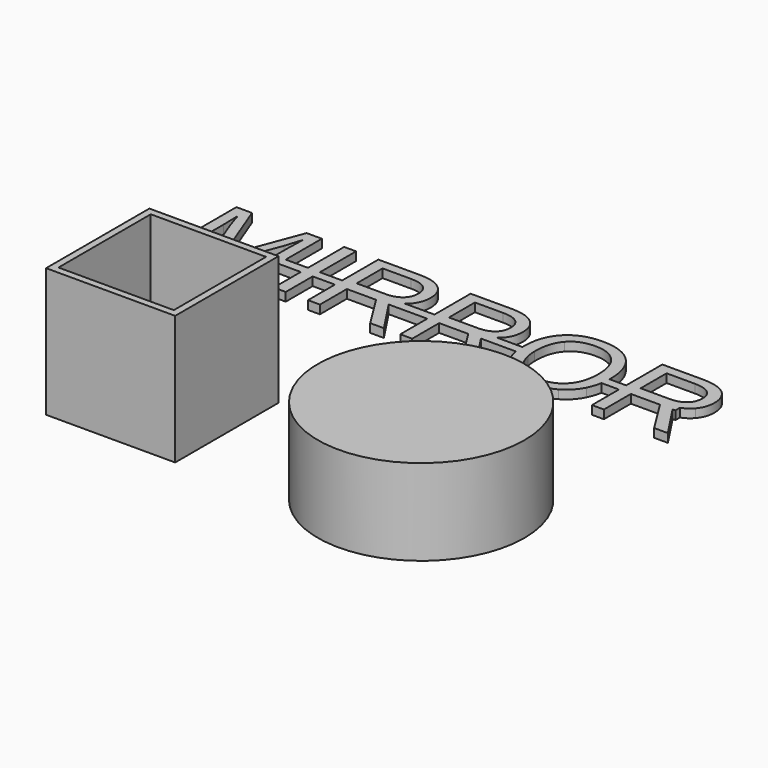
from build123d import *

# Parameters (mm, degrees)
F0_W     = 15
F0_H     = 15
F0_W_2   = 13.4
F0_H_2   = 13.4
F1_DEPTH = 15
F2_R     = 12
F3_DEPTH = 10
F4_W     = 0.2576843763
F4_H     = 1.0465048254
F4_W_2   = 1.2318606096
F4_H_2   = 3.9146672934
F4_W_3   = 1.2457799385
F4_W_4   = 2.5889951794
F4_W_5   = 1.3849732277
F4_H_3   = 5.2532954214
F4_W_6   = 2.5866752912
F5_DEPTH = 1


with BuildPart() as f1:
    # F0 (on Top) → F1 (new body)
    with BuildSketch(Plane.XY):
        with Locations((-3.6360850185, -0.7159802735)):
            Rectangle(F0_W, F0_H)
        with Locations((-3.6360850185, -0.7159802735)):
            Rectangle(F0_W_2, F0_H_2, mode=Mode.SUBTRACT)
    extrude(amount=F1_DEPTH)


with BuildPart() as f3:
    # F2 (on Top) → F3 (new body)
    with BuildSketch(Plane.XY):
        with Locations((25.8726727164, 0)):
            Circle(F2_R)
    extrude(amount=F3_DEPTH)


with BuildPart() as f5:
    # F4 (on Top) → F5 (new body)
    with BuildSketch(Plane.XY):
        with Locations((-22.0726660955, 27.1542668343)):
            Rectangle(F4_W, F4_H)
        Polygon((-21.9438239073, 32.9308146684), (-21.9438239073, 27.6775192469), (-20.7119632978, 27.6775192469), (-20.7119632978, 29.5321785234), (-20.7398019556, 30.900912534), (-20.7630008372, 31.7059137233), (-20.5217324692, 30.9078721984), (-20.1157520423, 29.6760115889), (-19.3476648189, 27.6775192469), (-18.1083718393, 27.6775192469), (-20.1250315949, 32.9308146684), align=None)
        with Locations((-21.3278936026, 27.1542668343)):
            Rectangle(F4_W_2, F4_H)
        Polygon((-19.3476648189, 27.6775192469), (-20.7119632978, 27.6775192469), (-20.7119632978, 26.6310144216), (-18.945458131, 26.6310144216), align=None)
        with Locations((-21.3278936026, 24.6736807749)):
            Rectangle(F4_W_2, F4_H_2)
        Polygon((-18.1083718393, 27.6775192469), (-19.3476648189, 27.6775192469), (-18.945458131, 26.6310144216), (-17.7066346447, 26.6310144216), align=None)
        Polygon((-15.7659015271, 27.6775192469), (-18.1083718393, 27.6775192469), (-17.7066346447, 26.6310144216), (-16.1600975799, 26.6310144216), align=None)
        with BuildLine():
            Line((-17.7066346447, 26.6310144216), (-18.945458131, 26.6310144216))
            Line((-18.945458131, 26.6310144216), (-17.4409210013, 22.7163471282))
            Line((-17.4409210013, 22.7163471282), (-16.4712077531, 22.7163471282))
            Line((-16.4712077531, 22.7163471282), (-14.9862439597, 26.6310144216))
            Line((-14.9862439597, 26.6310144216), (-16.1600975799, 26.6310144216))
            Line((-16.1600975799, 26.6310144216), (-16.454968536, 25.8481961355))
            add(Edge.make_bspline(
                [(-16.7055164566, 25.1046719823), (-16.5199254043, 25.6950835173), (-16.454968536, 25.8481961355)],
                knots=[0, 0, 0, 1, 1, 1], degree=2))
            add(Edge.make_bspline(
                [(-16.9491047127, 24.224274428), (-16.8911075089, 24.5142604472), (-16.7055164566, 25.1046719823)],
                knots=[0, 0, 0, 1, 1, 1], degree=2))
            add(Edge.make_bspline(
                [(-17.1265761564, 24.9318403148), (-16.9931825876, 24.4423439144), (-16.9491047127, 24.224274428)],
                knots=[0, 0, 0, 1, 1, 1], degree=2))
            add(Edge.make_bspline(
                [(-17.4061226789, 25.8481961355), (-17.2599697253, 25.4213367152), (-17.1265761564, 24.9318403148)],
                knots=[0, 0, 0, 1, 1, 1], degree=2))
            Line((-17.4061226789, 25.8481961355), (-17.7066346447, 26.6310144216))
        make_face()
        with BuildLine():
            Line((-13.7870971594, 32.9308146684), (-15.7659015271, 27.6775192469))
            Line((-15.7659015271, 27.6775192469), (-14.589269796, 27.6775192469))
            Line((-14.589269796, 27.6775192469), (-13.8311750343, 29.6760115889))
            add(Edge.make_bspline(
                [(-13.193205792, 31.7059137233), (-13.5481486795, 30.4090962454), (-13.8311750343, 29.6760115889)],
                knots=[0, 0, 0, 1, 1, 1], degree=2))
            add(Edge.make_bspline(
                [(-13.2581626603, 29.5321785234), (-13.2581626603, 30.6619640542), (-13.193205792, 31.7059137233)],
                knots=[0, 0, 0, 1, 1, 1], degree=2))
            Line((-13.2581626603, 29.5321785234), (-13.2581626603, 27.6775192469))
            Line((-13.2581626603, 27.6775192469), (-12.0123827219, 27.6775192469))
            Line((-12.0123827219, 27.6775192469), (-12.0123827219, 32.9308146684))
            Line((-12.0123827219, 32.9308146684), (-13.7870971594, 32.9308146684))
        make_face()
        Polygon((-14.589269796, 27.6775192469), (-15.7659015271, 27.6775192469), (-16.1600975799, 26.6310144216), (-14.9862439597, 26.6310144216), align=None)
        Polygon((-13.2581626603, 27.6775192469), (-14.589269796, 27.6775192469), (-14.9862439597, 26.6310144216), (-13.2581626603, 26.6310144216), align=None)
        with Locations((-12.6352726911, 27.1542668343)):
            Rectangle(F4_W_3, F4_H)
        with Locations((-10.7178851322, 27.1542668343)):
            Rectangle(F4_W_4, F4_H)
        with Locations((-12.6352726911, 24.6736807749)):
            Rectangle(F4_W_3, F4_H_2)
        with Locations((-8.7309009286, 30.3041669576)):
            Rectangle(F4_W_5, F4_H_3)
        with Locations((-8.7309009286, 27.1542668343)):
            Rectangle(F4_W_5, F4_H)
        with Locations((-6.7450766692, 27.1542668343)):
            Rectangle(F4_W_6, F4_H)
        with Locations((-8.7309009286, 24.6736807749)):
            Rectangle(F4_W_5, F4_H_2)
        with BuildLine():
            Line((-5.4517390236, 32.9308146684), (-5.4517390236, 27.6775192469))
            Line((-5.4517390236, 27.6775192469), (1.8461499898, 27.6775192469))
            add(Edge.make_bspline(
                [(2.2943675212, 28.0950078122), (2.0933608592, 27.8599143561), (1.8461499898, 27.6775192469)],
                knots=[0, 0, 0, 0.3029544746, 0.3029544746, 0.3029544746], degree=2))
            add(Edge.make_bspline(
                [(2.9578555332, 30.010075483), (2.9578555332, 28.8710103996), (2.2943675212, 28.0950078122)],
                knots=[0, 0, 0, 1, 1, 1], degree=2))
            add(Edge.make_bspline(
                [(2.019460775, 32.1594518573), (2.9578555332, 31.3880890462), (2.9578555332, 30.010075483)],
                knots=[0, 0, 0, 1, 1, 1], degree=2))
            add(Edge.make_bspline(
                [(-0.6449307693, 32.9308146684), (1.0810660169, 32.9308146684), (2.019460775, 32.1594518573)],
                knots=[0, 0, 0, 1, 1, 1], degree=2))
            Line((-0.6449307693, 32.9308146684), (-5.4517390236, 32.9308146684))
        make_face()
        with BuildLine():
            add(Edge.make_bspline(
                [(1.565922641, 29.9961561541), (1.565922641, 30.8869932051), (0.9604318329, 31.354450668)],
                knots=[0, 0, 0, 1, 1, 1], degree=2))
            add(Edge.make_bspline(
                [(0.9673914974, 28.5636252192), (1.565922641, 29.0751605571), (1.565922641, 29.9961561541)],
                knots=[0, 0, 0, 1, 1, 1], degree=2))
            add(Edge.make_bspline(
                [(-0.7238069666, 28.0520898814), (0.3688603538, 28.0520898814), (0.9673914974, 28.5636252192)],
                knots=[0, 0, 0, 1, 1, 1], degree=2))
            Line((-0.7238069666, 28.0520898814), (-4.0667657959, 28.0520898814))
            Line((-4.0667657959, 28.0520898814), (-4.0667657959, 31.821908131))
            Line((-4.0667657959, 31.821908131), (-0.7818041704, 31.821908131))
            add(Edge.make_bspline(
                [(0.9604318329, 31.354450668), (0.3549410249, 31.821908131), (-0.7818041704, 31.821908131)],
                knots=[0, 0, 0, 1, 1, 1], degree=2))
        make_face(mode=Mode.SUBTRACT)
        with BuildLine():
            Line((1.8461499898, 27.6775192469), (-5.4517390236, 27.6775192469))
            Line((-5.4517390236, 27.6775192469), (-5.4517390236, 26.6310144216))
            Line((-5.4517390236, 26.6310144216), (-4.0667657959, 26.6310144216))
            Line((-4.0667657959, 26.6310144216), (-4.0667657959, 26.9571026729))
            Line((-4.0667657959, 26.9571026729), (-0.8838792492, 26.9571026729))
            Line((-0.8838792492, 26.9571026729), (-0.6798065142, 26.6310144216))
            Line((-0.6798065142, 26.6310144216), (0.7843240376, 26.6310144216))
            Line((0.7843240376, 26.6310144216), (0.4639757681, 27.1171749555))
            add(Edge.make_bspline(
                [(1.8461499898, 27.6775192469), (1.2773607994, 27.2578598416), (0.4639757681, 27.1171749555)],
                knots=[0.3029544746, 0.3029544746, 0.3029544746, 1, 1, 1], degree=2))
        make_face()
        with BuildLine():
            Line((5.2707840223, 27.6775192469), (1.8461499898, 27.6775192469))
            add(Edge.make_bspline(
                [(1.8461499898, 27.6775192469), (1.2773607994, 27.2578598416), (0.4639757681, 27.1171749555)],
                knots=[0.3029544746, 0.3029544746, 0.3029544746, 1, 1, 1], degree=2))
            Line((0.4639757681, 27.1171749555), (0.7843240376, 26.6310144216))
            Line((0.7843240376, 26.6310144216), (5.2707840223, 26.6310144216))
            Line((5.2707840223, 26.6310144216), (5.2707840223, 27.6775192469))
        make_face()
        with Locations((-4.7592524097, 24.6736807749)):
            Rectangle(F4_W_5, F4_H_2)
        with BuildLine():
            Line((5.2707840223, 32.9308146684), (5.2707840223, 27.6775192469))
            Line((5.2707840223, 27.6775192469), (12.5686730356, 27.6775192469))
            add(Edge.make_bspline(
                [(13.0168905671, 28.0950078122), (12.815883905, 27.8599143561), (12.5686730356, 27.6775192469)],
                knots=[0, 0, 0, 0.3029544746, 0.3029544746, 0.3029544746], degree=2))
            add(Edge.make_bspline(
                [(13.680378579, 30.010075483), (13.680378579, 28.8710103996), (13.0168905671, 28.0950078122)],
                knots=[0, 0, 0, 1, 1, 1], degree=2))
            add(Edge.make_bspline(
                [(12.7419838209, 32.1594518573), (13.680378579, 31.3880890462), (13.680378579, 30.010075483)],
                knots=[0, 0, 0, 1, 1, 1], degree=2))
            add(Edge.make_bspline(
                [(10.0775922765, 32.9308146684), (11.8035890628, 32.9308146684), (12.7419838209, 32.1594518573)],
                knots=[0, 0, 0, 1, 1, 1], degree=2))
            Line((10.0775922765, 32.9308146684), (5.2707840223, 32.9308146684))
        make_face()
        with BuildLine():
            add(Edge.make_bspline(
                [(12.2884456869, 29.9961561541), (12.2884456869, 30.8869932051), (11.6829548788, 31.354450668)],
                knots=[0, 0, 0, 1, 1, 1], degree=2))
            add(Edge.make_bspline(
                [(11.6899145432, 28.5636252192), (12.2884456869, 29.0751605571), (12.2884456869, 29.9961561541)],
                knots=[0, 0, 0, 1, 1, 1], degree=2))
            add(Edge.make_bspline(
                [(9.9987160793, 28.0520898814), (11.0913833996, 28.0520898814), (11.6899145432, 28.5636252192)],
                knots=[0, 0, 0, 1, 1, 1], degree=2))
            Line((9.9987160793, 28.0520898814), (6.65575725, 28.0520898814))
            Line((6.65575725, 28.0520898814), (6.65575725, 31.821908131))
            Line((6.65575725, 31.821908131), (9.9407188754, 31.821908131))
            add(Edge.make_bspline(
                [(11.6829548788, 31.354450668), (11.0774640707, 31.821908131), (9.9407188754, 31.821908131)],
                knots=[0, 0, 0, 1, 1, 1], degree=2))
        make_face(mode=Mode.SUBTRACT)
        with BuildLine():
            Line((12.5686730356, 27.6775192469), (5.2707840223, 27.6775192469))
            Line((5.2707840223, 27.6775192469), (5.2707840223, 26.6310144216))
            Line((5.2707840223, 26.6310144216), (6.65575725, 26.6310144216))
            Line((6.65575725, 26.6310144216), (6.65575725, 26.9571026729))
            Line((6.65575725, 26.9571026729), (9.8386437967, 26.9571026729))
            Line((9.8386437967, 26.9571026729), (10.0427165316, 26.6310144216))
            Line((10.0427165316, 26.6310144216), (11.5068470835, 26.6310144216))
            Line((11.5068470835, 26.6310144216), (11.1864988139, 27.1171749555))
            add(Edge.make_bspline(
                [(12.5686730356, 27.6775192469), (11.9998838453, 27.2578598416), (11.1864988139, 27.1171749555)],
                knots=[0.3029544746, 0.3029544746, 0.3029544746, 1, 1, 1], degree=2))
        make_face()
        Polygon((-4.0667657959, 26.9571026729), (-4.0667657959, 26.6310144216), (-0.6798065142, 26.6310144216), (-0.8838792492, 26.9571026729), align=None)
        with BuildLine():
            Line((15.4805019964, 27.6775192469), (12.5686730356, 27.6775192469))
            add(Edge.make_bspline(
                [(12.5686730356, 27.6775192469), (11.9998838453, 27.2578598416), (11.1864988139, 27.1171749555)],
                knots=[0.3029544746, 0.3029544746, 0.3029544746, 1, 1, 1], degree=2))
            Line((11.1864988139, 27.1171749555), (11.5068470835, 26.6310144216))
            Line((11.5068470835, 26.6310144216), (15.5774134707, 26.6310144216))
            add(Edge.make_bspline(
                [(15.5774134707, 26.6310144216), (15.4930928582, 27.1302187098), (15.4805019964, 27.6775192469)],
                knots=[0.594228176, 0.594228176, 0.594228176, 0.9394096317, 0.9394096317, 0.9394096317], degree=2))
        make_face()
        with Locations((5.9632706361, 24.6736807749)):
            Rectangle(F4_W_5, F4_H_2)
        Polygon((3.36383596, 22.7163471282), (0.7843240376, 26.6310144216), (-0.6798065142, 26.6310144216), (1.7700727985, 22.7163471282), align=None)
        with BuildLine():
            add(Edge.make_bspline(
                [(15.4805019964, 27.6775192469), (15.478291898, 27.7735879684), (15.478291898, 27.8711386054)],
                knots=[0.9394096317, 0.9394096317, 0.9394096317, 1, 1, 1], degree=2))
            Line((15.4805019964, 27.6775192469), (16.886656882, 27.6775192469))
            add(Edge.make_bspline(
                [(16.8841441191, 27.8711386054), (16.8841441191, 27.7732997466), (16.886656882, 27.6775192469)],
                knots=[0, 0, 0, 0.0509347284, 0.0509347284, 0.0509347284], degree=2))
            add(Edge.make_bspline(
                [(17.8410979825, 30.8788735965), (16.8841441191, 29.8059253255), (16.8841441191, 27.8711386054)],
                knots=[0, 0, 0, 1, 1, 1], degree=2))
            add(Edge.make_bspline(
                [(20.5542071781, 31.9518218676), (18.7980518458, 31.9518218676), (17.8410979825, 30.8788735965)],
                knots=[0, 0, 0, 1, 1, 1], degree=2))
            add(Edge.make_bspline(
                [(23.2475973244, 30.8649542676), (22.2941232932, 31.9518218676), (20.5542071781, 31.9518218676)],
                knots=[0, 0, 0, 1, 1, 1], degree=2))
            add(Edge.make_bspline(
                [(24.2010713555, 27.8711386054), (24.2010713555, 29.7780866676), (23.2475973244, 30.8649542676)],
                knots=[0, 0, 0, 1, 1, 1], degree=2))
            add(Edge.make_bspline(
                [(24.1987870848, 27.6775192469), (24.2010713555, 27.7732413782), (24.2010713555, 27.8711386054)],
                knots=[0.9508741384, 0.9508741384, 0.9508741384, 1, 1, 1], degree=2))
            Line((24.1987870848, 27.6775192469), (25.6116152515, 27.6775192469))
            add(Edge.make_bspline(
                [(25.613883241, 27.8711386054), (25.613883241, 27.7735879637), (25.6116152515, 27.6775192469)],
                knots=[0, 0, 0, 0.0608534263, 0.0608534263, 0.0608534263], degree=2))
            add(Edge.make_bspline(
                [(25.0083924329, 30.6619640542), (25.613883241, 29.481140984), (25.613883241, 27.8711386054)],
                knots=[0, 0, 0, 1, 1, 1], degree=2))
            add(Edge.make_bspline(
                [(23.2580368211, 32.4633572054), (24.4029016249, 31.8427871243), (25.0083924329, 30.6619640542)],
                knots=[0, 0, 0, 1, 1, 1], degree=2))
            add(Edge.make_bspline(
                [(20.5542071781, 33.0839272865), (22.1131720173, 33.0839272865), (23.2580368211, 32.4633572054)],
                knots=[0, 0, 0, 1, 1, 1], degree=2))
            add(Edge.make_bspline(
                [(16.8191872508, 31.702433891), (18.1600826036, 33.0839272865), (20.5542071781, 33.0839272865)],
                knots=[0, 0, 0, 1, 1, 1], degree=2))
            add(Edge.make_bspline(
                [(15.478291898, 27.8711386054), (15.478291898, 30.3209404956), (16.8191872508, 31.702433891)],
                knots=[0, 0, 0, 1, 1, 1], degree=2))
        make_face()
        with BuildLine():
            Line((16.886656882, 27.6775192469), (15.4805019964, 27.6775192469))
            add(Edge.make_bspline(
                [(15.5774134707, 26.6310144216), (15.4930928582, 27.1302187098), (15.4805019964, 27.6775192469)],
                knots=[0.594228176, 0.594228176, 0.594228176, 0.9394096317, 0.9394096317, 0.9394096317], degree=2))
            Line((15.5774134707, 26.6310144216), (17.0012932481, 26.6310144216))
            add(Edge.make_bspline(
                [(16.886656882, 27.6775192469), (16.9013012747, 27.1193101006), (17.0012932481, 26.6310144216)],
                knots=[0.0509347284, 0.0509347284, 0.0509347284, 0.3477825348, 0.3477825348, 0.3477825348], degree=2))
        make_face()
        Polygon((6.65575725, 26.9571026729), (6.65575725, 26.6310144216), (10.0427165316, 26.6310144216), (9.8386437967, 26.9571026729), align=None)
        with BuildLine():
            Line((17.0012932481, 26.6310144216), (15.5774134707, 26.6310144216))
            add(Edge.make_bspline(
                [(16.0803028739, 25.054794387), (15.7225709898, 25.7716366981), (15.5774134707, 26.6310144216)],
                knots=[0, 0, 0, 0.594228176, 0.594228176, 0.594228176], degree=2))
            add(Edge.make_bspline(
                [(17.8236988213, 23.2093233608), (16.6823138497, 23.8484525471), (16.0803028739, 25.054794387)],
                knots=[0, 0, 0, 1, 1, 1], degree=2))
            add(Edge.make_bspline(
                [(20.537967961, 22.5701941745), (18.9650837929, 22.5701941745), (17.8236988213, 23.2093233608)],
                knots=[0, 0, 0, 1, 1, 1], degree=2))
            add(Edge.make_bspline(
                [(23.2429575481, 23.2162830252), (22.0969328002, 22.5701941745), (20.537967961, 22.5701941745)],
                knots=[0, 0, 0, 1, 1, 1], degree=2))
            add(Edge.make_bspline(
                [(25.0014327685, 25.0652338837), (24.3889822959, 23.862371876), (23.2429575481, 23.2162830252)],
                knots=[0, 0, 0, 1, 1, 1], degree=2))
            add(Edge.make_bspline(
                [(25.5121652205, 26.6310144216), (25.3642890709, 25.7778891595), (25.0014327685, 25.0652338837)],
                knots=[0.4075336395, 0.4075336395, 0.4075336395, 1, 1, 1], degree=2))
            Line((25.5121652205, 26.6310144216), (24.093700339, 26.6310144216))
            add(Edge.make_bspline(
                [(23.2545569888, 24.7868473052), (23.8822795587, 25.510728357), (24.093700339, 26.6310144216)],
                knots=[0, 0, 0, 0.6631939165, 0.6631939165, 0.6631939165], degree=2))
            add(Edge.make_bspline(
                [(20.537967961, 23.695339929), (22.3080426222, 23.695339929), (23.2545569888, 24.7868473052)],
                knots=[0, 0, 0, 1, 1, 1], degree=2))
            add(Edge.make_bspline(
                [(17.8526974232, 24.8228055716), (18.8212507273, 23.695339929), (20.537967961, 23.695339929)],
                knots=[0, 0, 0, 1, 1, 1], degree=2))
            add(Edge.make_bspline(
                [(17.0012932481, 26.6310144216), (17.2209900423, 25.5581583551), (17.8526974232, 24.8228055716)],
                knots=[0.3477825348, 0.3477825348, 0.3477825348, 1, 1, 1], degree=2))
        make_face()
        Polygon((14.0863590059, 22.7163471282), (11.5068470835, 26.6310144216), (10.0427165316, 26.6310144216), (12.4925958444, 22.7163471282), align=None)
        with BuildLine():
            Line((25.6116152515, 27.6775192469), (24.1987870848, 27.6775192469))
            add(Edge.make_bspline(
                [(24.093700339, 26.6310144216), (24.1854104338, 27.1169720512), (24.1987870848, 27.6775192469)],
                knots=[0.6631939165, 0.6631939165, 0.6631939165, 0.9508741384, 0.9508741384, 0.9508741384], degree=2))
            Line((24.093700339, 26.6310144216), (25.5121652205, 26.6310144216))
            add(Edge.make_bspline(
                [(25.6116152515, 27.6775192469), (25.5986945806, 27.1302185409), (25.5121652205, 26.6310144216)],
                knots=[0.0608534263, 0.0608534263, 0.0608534263, 0.4075336395, 0.4075336395, 0.4075336395], degree=2))
        make_face()
        with BuildLine():
            Line((27.5417102966, 27.6775192469), (25.6116152515, 27.6775192469))
            add(Edge.make_bspline(
                [(25.6116152515, 27.6775192469), (25.5986945806, 27.1302185409), (25.5121652205, 26.6310144216)],
                knots=[0.0608534263, 0.0608534263, 0.0608534263, 0.4075336395, 0.4075336395, 0.4075336395], degree=2))
            Line((25.5121652205, 26.6310144216), (27.5417102966, 26.6310144216))
            Line((27.5417102966, 26.6310144216), (27.5417102966, 27.6775192469))
        make_face()
        with BuildLine():
            Line((27.5417102966, 32.9308146684), (27.5417102966, 27.6775192469))
            Line((27.5417102966, 27.6775192469), (34.0978913009, 27.6775192469))
            Line((34.0978913009, 27.6775192469), (34.0978913009, 27.2846954567))
            add(Edge.make_bspline(
                [(35.2878168414, 28.0950078122), (34.8186912314, 27.5463276844), (34.0978913009, 27.2846954567)],
                knots=[0, 0, 0, 0.7070596629, 0.7070596629, 0.7070596629], degree=2))
            add(Edge.make_bspline(
                [(35.9513048534, 30.010075483), (35.9513048534, 28.8710103996), (35.2878168414, 28.0950078122)],
                knots=[0, 0, 0, 1, 1, 1], degree=2))
            add(Edge.make_bspline(
                [(35.0129100952, 32.1594518573), (35.9513048534, 31.3880890462), (35.9513048534, 30.010075483)],
                knots=[0, 0, 0, 1, 1, 1], degree=2))
            add(Edge.make_bspline(
                [(32.3485185509, 32.9308146684), (34.0745153371, 32.9308146684), (35.0129100952, 32.1594518573)],
                knots=[0, 0, 0, 1, 1, 1], degree=2))
            Line((32.3485185509, 32.9308146684), (27.5417102966, 32.9308146684))
        make_face()
        with BuildLine():
            add(Edge.make_bspline(
                [(34.5593719612, 29.9961561541), (34.5593719612, 30.8869932051), (33.9538811531, 31.354450668)],
                knots=[0, 0, 0, 1, 1, 1], degree=2))
            add(Edge.make_bspline(
                [(33.9608408176, 28.5636252192), (34.5593719612, 29.0751605571), (34.5593719612, 29.9961561541)],
                knots=[0, 0, 0, 1, 1, 1], degree=2))
            add(Edge.make_bspline(
                [(32.2696423536, 28.0520898814), (33.362309674, 28.0520898814), (33.9608408176, 28.5636252192)],
                knots=[0, 0, 0, 1, 1, 1], degree=2))
            Line((32.2696423536, 28.0520898814), (28.9266835243, 28.0520898814))
            Line((28.9266835243, 28.0520898814), (28.9266835243, 31.821908131))
            Line((28.9266835243, 31.821908131), (32.2116451498, 31.821908131))
            add(Edge.make_bspline(
                [(33.9538811531, 31.354450668), (33.3483903451, 31.821908131), (32.2116451498, 31.821908131)],
                knots=[0, 0, 0, 1, 1, 1], degree=2))
        make_face(mode=Mode.SUBTRACT)
        with BuildLine():
            Line((34.0978913009, 27.6775192469), (27.5417102966, 27.6775192469))
            Line((27.5417102966, 27.6775192469), (27.5417102966, 26.6310144216))
            Line((27.5417102966, 26.6310144216), (28.9266835243, 26.6310144216))
            Line((28.9266835243, 26.6310144216), (28.9266835243, 26.9571026729))
            Line((28.9266835243, 26.9571026729), (32.109570071, 26.9571026729))
            Line((32.109570071, 26.9571026729), (32.313642806, 26.6310144216))
            Line((32.313642806, 26.6310144216), (33.7777733578, 26.6310144216))
            Line((33.7777733578, 26.6310144216), (33.4574250883, 27.1171749555))
            add(Edge.make_bspline(
                [(34.0978913009, 27.2846954567), (33.7992582636, 27.1762991826), (33.4574250883, 27.1171749555)],
                knots=[0.7070596629, 0.7070596629, 0.7070596629, 1, 1, 1], degree=2))
            Line((34.0978913009, 27.2846954567), (34.0978913009, 27.6775192469))
        make_face()
        with Locations((28.2341969105, 24.6736807749)):
            Rectangle(F4_W_5, F4_H_2)
        with BuildLine():
            Line((34.0978913009, 26.6310144216), (34.0978913009, 27.2846954567))
            add(Edge.make_bspline(
                [(34.0978913009, 27.2846954567), (33.7992582636, 27.1762991826), (33.4574250883, 27.1171749555)],
                knots=[0.7070596629, 0.7070596629, 0.7070596629, 1, 1, 1], degree=2))
            Line((33.4574250883, 27.1171749555), (33.7777733578, 26.6310144216))
            Line((33.7777733578, 26.6310144216), (34.0978913009, 26.6310144216))
        make_face()
        Polygon((28.9266835243, 26.9571026729), (28.9266835243, 26.6310144216), (32.313642806, 26.6310144216), (32.109570071, 26.9571026729), align=None)
        Polygon((33.7777733578, 26.6310144216), (32.313642806, 26.6310144216), (34.7635221187, 22.7163471282), (36.3572852802, 22.7163471282), align=None)
    extrude(amount=F5_DEPTH)


solid = Compound([f1.part, f3.part, f5.part])
